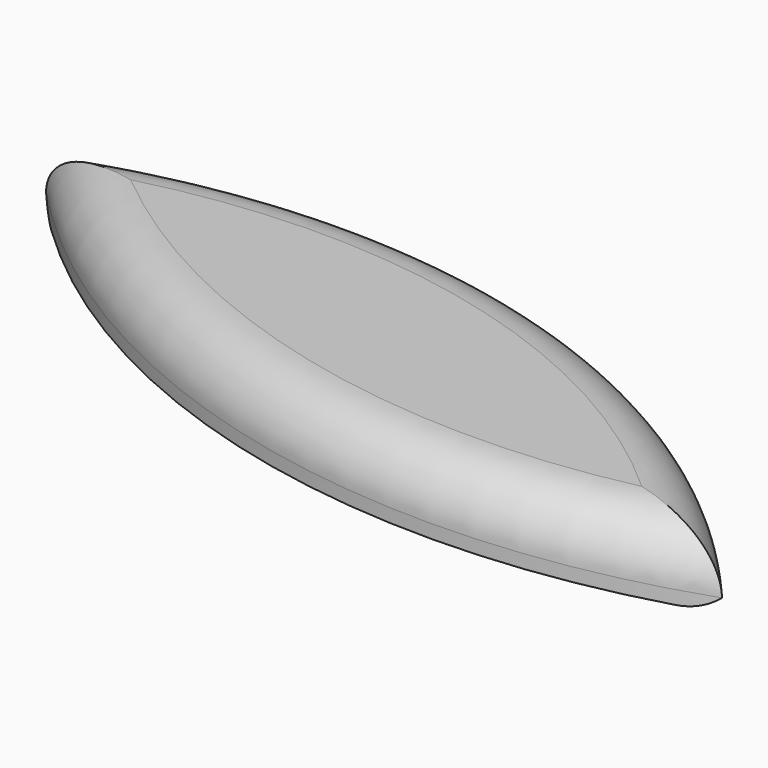
from build123d import *

# Parameters (mm, degrees)
F1_DEPTH    = 6.35
F2_R        = 5.08
F3_T2_ANGLE = 84.7300035824


# Not quite as in the source:
# - a fillet or chamfer that OpenCascade refuses, or shapes differently, is made with other operations: its cross-section is extruded or revolved along the edge and cut away or added


with BuildPart() as f1:
    # F0 (on Top) → F1 (new body)
    with BuildSketch(Plane.XY):
        with BuildLine():
            ThreePointArc((-58.4820285439, 30.5738802999), (-95.0022427224, 52.9656761429), (-137.7363353968, 49.9797277153))
            ThreePointArc((-137.7363353968, 49.9797277153), (-100.9651889281, 28.6127500264), (-58.4820285439, 30.5738802999))
        make_face()
    extrude(amount=F1_DEPTH)

    # F2
    f2_edges = [f1.edges().sort_by_distance(p)[0] for p in [
        (-100.965189, 28.61275, 6.35),
        (-95.002243, 52.965676, 6.35),
    ]]
    fillet(f2_edges, radius=F2_R)

    # F3: fillet of radius 5.08 on 2 edges, made by hand

    # F3_s1 → F3_t2 (revolve, cut)
    with BuildSketch(Plane(origin=(-27.6470070166, 41.1795425882, 0), x_dir=(0, 0, 1), z_dir=(0.557404804, -0.8302408593, 0))):
        with BuildLine():
            ThreePointArc((1.27, 31.0101609977), (0.3280951188, 32.5742139386), (0, 34.3702651628))
            Line((0, 34.3702651628), (0, 31.0101609977))
            Line((0, 31.0101609977), (1.27, 31.0101609977))
        make_face()
    revolve(axis=Axis((-111.7067534455, -15.2562566767, 0), (0, 0, 1)), revolution_arc=F3_T2_ANGLE, mode=Mode.SUBTRACT)


solid = f1.part
